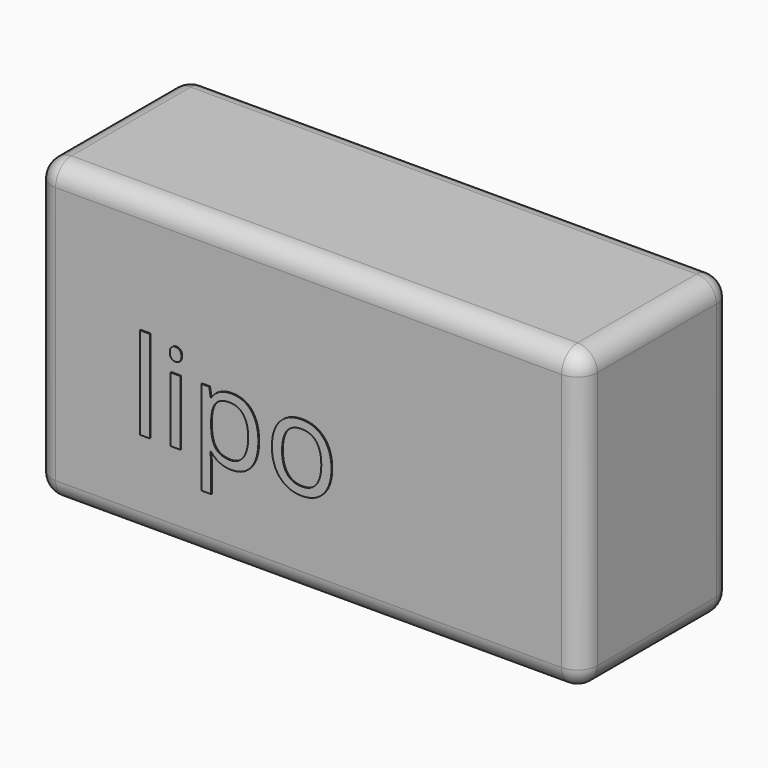
from build123d import *

# Parameters (mm, degrees)
F0_W         = 55
F0_H         = 30
F1_DEPTH     = 19
F2_R         = 2
F3_TEXT_SIZE = 12.2098006412
F4_DEPTH     = 0.1


# Not quite as in the source:
# - Text() gives the source's letters only with a copy of the font that has no kerning and outlines rounded to 1/6400 em; it was checked with that copy


with BuildPart() as f1:
    # F0 (on Front) → F1 (new body)
    with BuildSketch(Plane.XZ):
        with Locations((-34.1123342514, 17.5004121507)):
            Rectangle(F0_W, F0_H)
    extrude(amount=F1_DEPTH)

    # F2
    f2_edges = [f1.edges().sort_by_distance(p)[0] for p in [
        (-61.612334, -9.5, 32.500412),
        (-34.112334, -19, 32.500412),
        (-61.612334, -19, 17.500412),
        (-34.112334, -19, 2.500412),
        (-6.612334, -19, 17.500412),
        (-6.612334, 0, 17.500412),
        (-6.612334, -9.5, 32.500412),
        (-34.112334, 0, 32.500412),
        (-6.612334, -9.5, 2.500412),
        (-34.112334, 0, 2.500412),
        (-61.612334, -9.5, 2.500412),
        (-61.612334, 0, 17.500412),
    ]]
    fillet(f2_edges, radius=F2_R)

    # F3 (on face) → F4 (join)
    with BuildSketch(Plane.XZ.offset(19)):
        with Locations((-52.0757958293, 11.3948164508)):
            Text('lipo', F3_TEXT_SIZE, font='Open Sans', text_align=(TextAlign.LEFT, TextAlign.BOTTOM))
    extrude(amount=F4_DEPTH)


solid = f1.part
